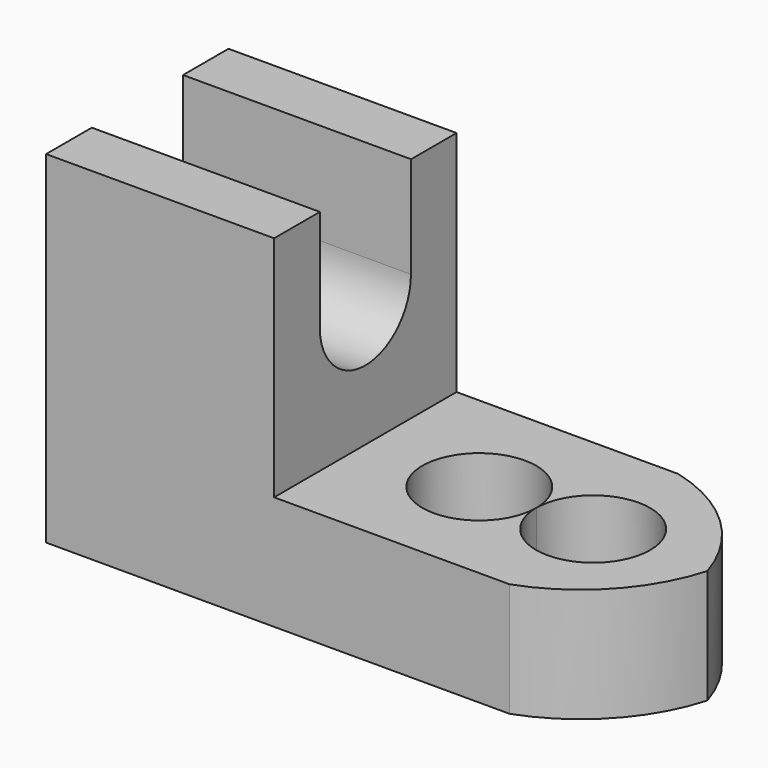
from build123d import *

# Parameters (mm, degrees)
F1_DEPTH = 25.4
F3_DEPTH = 25.4
F4_R     = 6.35
F5_DEPTH = 25.4
F6_R     = 6.35
F7_DEPTH = 25.401
F9_DEPTH = 25.4


# Not quite as in the source:
# - ends of sketch curves that miss each other by under 0.0002 mm in the source are joined


with BuildPart() as f1:
    # F0 (on Front) → F1 (new body)
    with BuildSketch(Plane.XZ):
        Polygon((-76.163366437, 49.151442945), (-76.163366437, 11.051442945), (-12.663366437, 11.051442945), (-12.663366437, 23.751442945), (-50.763366437, 23.751442945), (-50.763366437, 49.151442945), align=None)
    extrude(amount=F1_DEPTH)

    # F2 (on face) → F3 (cut)
    with BuildSketch(Plane.XY.offset(23.751442945)):
        with BuildLine():
            ThreePointArc((-26.0716341436, 0), (-17.7255959226, -4.6165280857), (-12.663366437, -12.7))
            Line((-12.663366437, -12.7), (-12.663366437, 0))
            Line((-12.663366437, 0), (-26.0716341436, 0))
        make_face()
        with BuildLine():
            Line((-12.663366437, -25.4), (-12.663366437, -12.7))
            ThreePointArc((-12.663366437, -12.7), (-17.065136592, -20.482800112), (-24.5329812169, -25.4))
            Line((-24.5329812169, -25.4), (-12.663366437, -25.4))
        make_face()
    extrude(amount=-F3_DEPTH, mode=Mode.SUBTRACT)

    # F4 (on face) → F5 (cut)
    with BuildSketch(Plane.XY.offset(23.751442945)):
        with BuildLine():
            ThreePointArc((-19.0133373642, -12.7271744008), (-25.3531445932, -6.3771825813), (-31.7133046421, -12.7067888852))
            ThreePointArc((-31.7133046421, -12.7067888852), (-25.3735301351, -19.0771662202), (-19.0133373642, -12.7271744008))
        make_face()
        with Locations((-38.0633682514, -12.706788681)):
            Circle(F4_R)
    extrude(amount=-F5_DEPTH, mode=Mode.SUBTRACT)

    # F6 (on face) → F7 (cut, through all)
    with BuildSketch(Plane.YZ.offset(-50.763366437)):
        with Locations((-12.7, 37.8679819405)):
            Circle(F6_R)
    extrude(amount=-F7_DEPTH, mode=Mode.SUBTRACT)

    # F8 (on face) → F9 (cut)
    with BuildSketch(Plane.YZ.offset(-50.763366437)):
        with BuildLine():
            Line((-19.0313366339, 49.151442945), (-19.0313366339, 38.3544759569))
            ThreePointArc((-19.0313366339, 38.3544759569), (-12.456574062, 44.2133143835), (-6.35, 37.8679819405))
            Line((-6.35, 37.8679819405), (-6.3313366339, 49.151442945))
            Line((-6.3313366339, 49.151442945), (-19.0313366339, 49.151442945))
        make_face()
    extrude(amount=-F9_DEPTH, mode=Mode.SUBTRACT)


solid = f1.part
